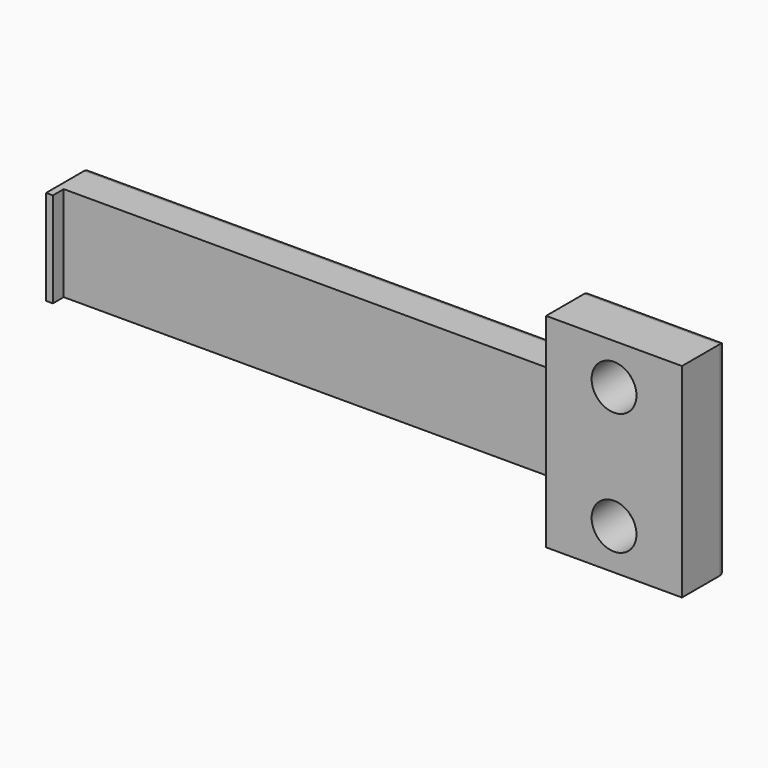
from build123d import *

# Parameters (mm, degrees)
F3_DEPTH       = 7
F5_DEPTH       = 4
F5_DEPTH_BACK  = 11
F7_D           = 3.3
F7_CSINK_D     = 5
F7_CSINK_ANGLE = 90
F8_T1_DEPTH    = 38.05
F8_T3_DEPTH    = 9.5
F8_T5_DEPTH    = 12.5
F8_T7_DEPTH    = 5.25
F8_T9_DEPTH    = 5.25
F8_T11_DEPTH   = 17.5
F8_T17_DEPTH   = 39.3
F8_T21_DEPTH   = 6.5
F8_T28_DEPTH   = 39.3
F8_T32_DEPTH   = 6.5


# Not quite as in the source:
# - a fillet or chamfer that OpenCascade refuses, or shapes differently, is made with other operations: its cross-section is extruded or revolved along the edge and cut away or added


with BuildPart() as f3:
    # F2 (on Top) → F3 (new body)
    with BuildSketch(Plane.XY):
        Polygon((0, 4), (0, 0), (0.5, 0), (0.5, 1), (36.8, 1), (36.8, 0), (46.8, 0), (46.8, 4), align=None)
    extrude(amount=F3_DEPTH)

    # F4 (on face) → F5 (join, two sides)
    with BuildSketch(Plane.XY.offset(7)) as f5_sk:
        Polygon((36.8, 1), (36.8, 0), (46.8, 0), (46.8, 4), (36.8, 4), align=None)
    extrude(amount=F5_DEPTH)
    extrude(f5_sk.sketch, amount=-F5_DEPTH_BACK)

    # F7 (through all)
    with Locations(Plane(origin=(0, 4, 0), x_dir=(-1, 0, 0), z_dir=(0, 1, 0))):
        with Locations((-41.8, 8), (-41.8, -1)):
            CounterSinkHole(F7_D / 2, F7_CSINK_D / 2, counter_sink_angle=F7_CSINK_ANGLE)

    # F8: fillet of radius 0.5 on 8 edges, made by hand

    # F8_s2 → F8_t1 (cut)
    with BuildSketch(Plane.YZ.offset(-1.25)):
        with BuildLine():
            ThreePointArc((4, 6.5), (3.8535533906, 6.8535533906), (3.5, 7))
            Line((3.5, 7), (4, 7))
            Line((4, 7), (4, 6.5))
        make_face()
        with BuildLine():
            ThreePointArc((4, 0.5), (3.8535533906, 0.1464466094), (3.5, 0))
            Line((3.5, 0), (4, 0))
            Line((4, 0), (4, 0.5))
        make_face()
    extrude(amount=F8_T1_DEPTH, mode=Mode.SUBTRACT)

    # F8_s4 → F8_t3 (cut)
    with BuildSketch(Plane.XY.offset(-1.25)):
        with BuildLine():
            ThreePointArc((0, 3.5), (0.1464466094, 3.8535533906), (0.5, 4))
            Line((0.5, 4), (0, 4))
            Line((0, 4), (0, 3.5))
        make_face()
    extrude(amount=F8_T3_DEPTH, mode=Mode.SUBTRACT)

    # F8_s6 → F8_t5 (cut)
    with BuildSketch(Plane.YZ.offset(35.55)):
        with BuildLine():
            ThreePointArc((4, -3.5), (3.8535533906, -3.8535533906), (3.5, -4))
            Line((3.5, -4), (4, -4))
            Line((4, -4), (4, -3.5))
        make_face()
        with BuildLine():
            ThreePointArc((4, 10.5), (3.8535533906, 10.8535533906), (3.5, 11))
            Line((3.5, 11), (4, 11))
            Line((4, 11), (4, 10.5))
        make_face()
    extrude(amount=F8_T5_DEPTH, mode=Mode.SUBTRACT)

    # F8_s8 → F8_t7 (cut)
    with BuildSketch(Plane.XY.offset(-5.25)):
        with BuildLine():
            ThreePointArc((37.3, 4), (36.9464466094, 3.8535533906), (36.8, 3.5))
            Line((36.8, 3.5), (36.8, 4))
            Line((36.8, 4), (37.3, 4))
        make_face()
    extrude(amount=F8_T7_DEPTH, mode=Mode.SUBTRACT)

    # F8_s10 → F8_t9 (cut)
    with BuildSketch(Plane.XY.offset(7)):
        with BuildLine():
            ThreePointArc((37.3, 4), (36.9464466094, 3.8535533906), (36.8, 3.5))
            Line((36.8, 3.5), (36.8, 4))
            Line((36.8, 4), (37.3, 4))
        make_face()
    extrude(amount=F8_T9_DEPTH, mode=Mode.SUBTRACT)

    # F8_s12 → F8_t11 (cut)
    with BuildSketch(Plane.XY.offset(-5.25)):
        with BuildLine():
            ThreePointArc((46.3, 4), (46.6535533906, 3.8535533906), (46.8, 3.5))
            Line((46.8, 3.5), (46.8, 4))
            Line((46.8, 4), (46.3, 4))
        make_face()
    extrude(amount=F8_T11_DEPTH, mode=Mode.SUBTRACT)


with BuildPart() as f8_tool15:
    # F8_s16 → F8_t17 (new body)
    with BuildSketch(Plane.YZ.offset(38.05)):
        with BuildLine():
            ThreePointArc((4, 6.5), (3.8535533906, 6.8535533906), (3.5, 7))
            Line((3.5, 7), (4, 7))
            Line((4, 7), (4, 6.5))
        make_face()
    extrude(amount=-F8_T17_DEPTH)

    split(bisect_by=Plane.YZ.offset(36.8), keep=Keep.TOP)


with BuildPart() as f8_tool19:
    # F8_s20 → F8_t21 (new body)
    with BuildSketch(Plane.XY.offset(12.25)):
        with BuildLine():
            ThreePointArc((37.3, 4), (36.9464466094, 3.8535533906), (36.8, 3.5))
            Line((36.8, 3.5), (36.8, 4))
            Line((36.8, 4), (37.3, 4))
        make_face()
    extrude(amount=-F8_T21_DEPTH)

    split(bisect_by=Plane.XY.offset(7), keep=Keep.BOTTOM)


with BuildPart() as f8_tool15_1:
    add(f8_tool15.part)

    # F8_t23: intersect F8_tool19
    add(f8_tool19.part, mode=Mode.INTERSECT)


with BuildPart() as f3_1:
    add(f3.part)

    # F8_t13: cut F8_tool15
    add(f8_tool15_1.part, mode=Mode.SUBTRACT)


with BuildPart() as f8_tool26:
    # F8_s27 → F8_t28 (new body)
    with BuildSketch(Plane.YZ.offset(38.05)):
        with BuildLine():
            ThreePointArc((4, 0.5), (3.8535533906, 0.1464466094), (3.5, 0))
            Line((3.5, 0), (4, 0))
            Line((4, 0), (4, 0.5))
        make_face()
    extrude(amount=-F8_T28_DEPTH)

    split(bisect_by=Plane.YZ.offset(36.8), keep=Keep.TOP)


with BuildPart() as f8_tool30:
    # F8_s31 → F8_t32 (new body)
    with BuildSketch(Plane.XY.offset(1.25)):
        with BuildLine():
            ThreePointArc((37.3, 4), (36.9464466094, 3.8535533906), (36.8, 3.5))
            Line((36.8, 3.5), (36.8, 4))
            Line((36.8, 4), (37.3, 4))
        make_face()
    extrude(amount=-F8_T32_DEPTH)

    split(bisect_by=Plane.XY, keep=Keep.TOP)


with BuildPart() as f8_tool26_1:
    add(f8_tool26.part)

    # F8_t34: intersect F8_tool30
    add(f8_tool30.part, mode=Mode.INTERSECT)


with BuildPart() as f3_2:
    add(f3_1.part)

    # F8_t24: cut F8_tool26
    add(f8_tool26_1.part, mode=Mode.SUBTRACT)


solid = f3_2.part
